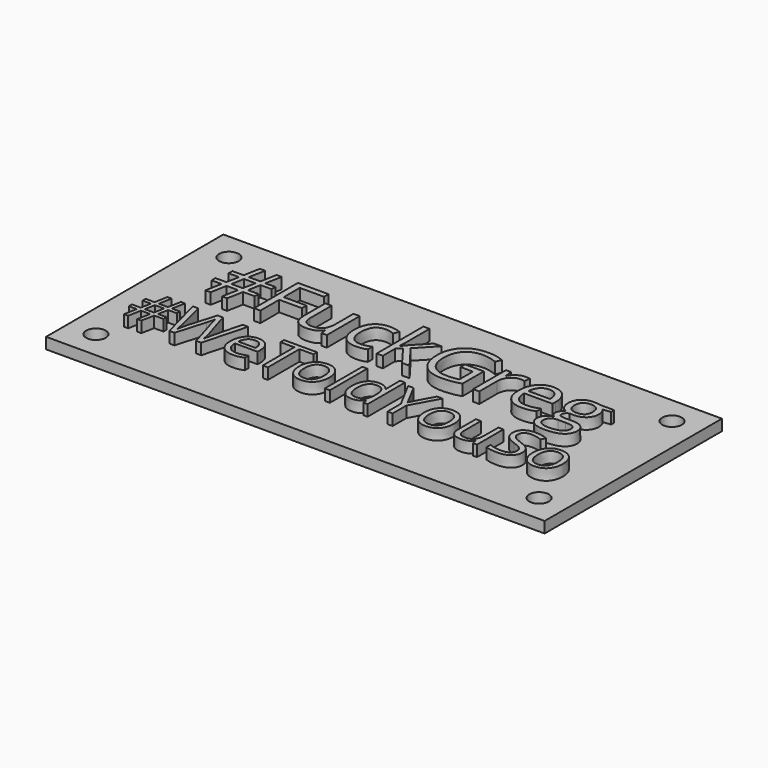
from build123d import *

# Parameters (mm, degrees)
F1_W           = 114.3
F1_H           = 50.8
F2_DEPTH       = 2.54
F0_TEXT_SIZE   = 17.6388888889
F0_TEXT_SIZE_2 = 14.1111111111
F3_DEPTH       = 2.54
F4_R           = 2.2479
F5_DEPTH       = 2.541


# Not quite as in the source:
# - Text() gives the source's letters only with a copy of the font that has no kerning and outlines rounded to 1/6400 em; it was checked with that copy


with BuildPart() as f2:
    # F1 (on Top) → F2 (new body)
    with BuildSketch(Plane.XY):
        with Locations((-57.15, 25.4)):
            Rectangle(F1_W, F1_H)
    extrude(amount=-F2_DEPTH)

    # F4 (on face) → F5 (cut, through all)
    with BuildSketch(Plane.XY):
        with Locations((-107.95, 44.45)):
            Circle(F4_R)
        with Locations((-6.35, 44.45)):
            Circle(F4_R)
        with Locations((-6.35, 6.35)):
            Circle(F4_R)
        with Locations((-107.95, 6.35)):
            Circle(F4_R)
    extrude(amount=-F5_DEPTH, mode=Mode.SUBTRACT)


with BuildPart() as f3:
    # F0 (on Top) → F3 (new body)
    with BuildSketch(Plane.XY):
        with Locations((-102.2219845712, 28.0840162516)):
            Text('#FuckGreg', F0_TEXT_SIZE, font='Open Sans', text_align=(TextAlign.LEFT, TextAlign.BOTTOM))
        with Locations((-107.4221950823, 11.7442273238)):
            Text('#WeToldYouSo', F0_TEXT_SIZE_2, font='Open Sans', text_align=(TextAlign.LEFT, TextAlign.BOTTOM))
    extrude(amount=F3_DEPTH)


solid = Compound([f2.part, f3.part])
